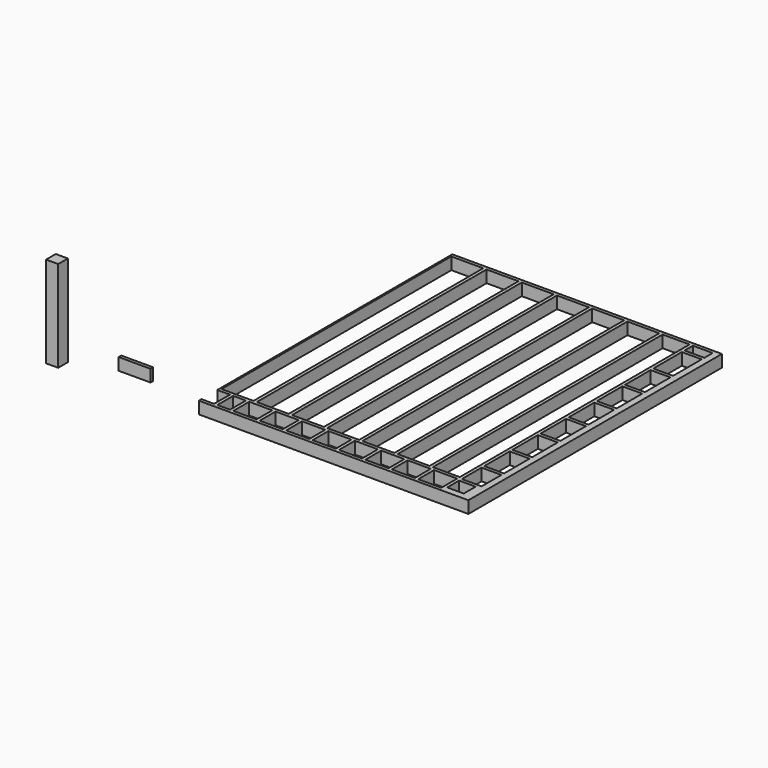
from build123d import *

# Parameters (mm, degrees)
F0_W     = 146.05
F0_H     = 228.6
F0_W_2   = 266.7
F0_W_3   = 190.5
F0_H_2   = 171.45
F0_W_4   = 228.6
F0_H_3   = 368.3
F0_W_5   = 368.3
F0_H_4   = 3314.7
F0_W_6   = 311.15
F0_H_5   = 412.75
F0_H_6   = 120.65
F1_DEPTH = 139.7
F2_W     = 139.7
F2_H     = 139.7
F3_DEPTH = 1054.1
F4_W     = 368.3
F4_H     = 139.7
F5_DEPTH = 38.1


# Not quite as in the source:
# - a feature names something its author has since deleted; it is built from what else it names


with BuildPart() as f1:
    # F0 (on Top) → F1 (new body)
    with BuildSketch(Plane.XY):
        Polygon((403.5037457943, 3406.0115362167), (-2669.8962542057, 3406.0115362167), (-2669.8962542057, 3367.9115362167), (-2669.8962542057, 53.2115362167), (-2669.8962542057, 15.1115362167), (-2523.8462542057, 15.1115362167), (-2523.8462542057, -213.4884637833), (-2669.8962542057, -213.4884637833), (-2669.8962542057, -251.5884637833), (403.5037457943, -251.5884637833), (441.6037457943, -251.5884637833), (441.6037457943, 3406.0115362167), align=None)
        with Locations((-2412.7212542057, -99.1884637833)):
            Rectangle(F0_W, F0_H, mode=Mode.SUBTRACT)
        with Locations((-2168.2462542057, -99.1884637833)):
            Rectangle(F0_W_2, F0_H, mode=Mode.SUBTRACT)
        with Locations((-1863.4462542057, -99.1884637833)):
            Rectangle(F0_W_2, F0_H, mode=Mode.SUBTRACT)
        with Locations((-1558.6462542057, -99.1884637833)):
            Rectangle(F0_W_2, F0_H, mode=Mode.SUBTRACT)
        with Locations((-1253.8462542057, -99.1884637833)):
            Rectangle(F0_W_2, F0_H, mode=Mode.SUBTRACT)
        with Locations((-949.0462542057, -99.1884637833)):
            Rectangle(F0_W_2, F0_H, mode=Mode.SUBTRACT)
        with Locations((-644.2462542057, -99.1884637833)):
            Rectangle(F0_W_2, F0_H, mode=Mode.SUBTRACT)
        with Locations((-339.4462542057, -99.1884637833)):
            Rectangle(F0_W_2, F0_H, mode=Mode.SUBTRACT)
        with Locations((-34.6462542057, -99.1884637833)):
            Rectangle(F0_W_2, F0_H, mode=Mode.SUBTRACT)
        with Locations((232.0537457943, -89.6634637833)):
            Rectangle(F0_W_3, F0_H_2, mode=Mode.SUBTRACT)
        Polygon((365.4037457943, 319.9115362167), (365.4037457943, 65.9115362167), (365.4037457943, 53.2115362167), (365.4037457943, 34.1615362167), (136.8037457943, 34.1615362167), (136.8037457943, 53.2115362167), (136.8037457943, 65.9115362167), (136.8037457943, 319.9115362167), align=None, mode=Mode.SUBTRACT)
        with Locations((251.1037457943, 542.1615362167)):
            Rectangle(F0_W_4, F0_H_3, mode=Mode.SUBTRACT)
        with Locations((251.1037457943, 948.5615362167)):
            Rectangle(F0_W_4, F0_H_3, mode=Mode.SUBTRACT)
        with Locations((251.1037457943, 1354.9615362167)):
            Rectangle(F0_W_4, F0_H_3, mode=Mode.SUBTRACT)
        with Locations((-2466.6962542057, 1710.5615362167)):
            Rectangle(F0_W_5, F0_H_4, mode=Mode.SUBTRACT)
        with Locations((-2060.2962542057, 1710.5615362167)):
            Rectangle(F0_W_5, F0_H_4, mode=Mode.SUBTRACT)
        with Locations((-1653.8962542057, 1710.5615362167)):
            Rectangle(F0_W_5, F0_H_4, mode=Mode.SUBTRACT)
        with Locations((-1247.4962542057, 1710.5615362167)):
            Rectangle(F0_W_5, F0_H_4, mode=Mode.SUBTRACT)
        with Locations((-841.0962542057, 1710.5615362167)):
            Rectangle(F0_W_5, F0_H_4, mode=Mode.SUBTRACT)
        with Locations((-434.6962542057, 1710.5615362167)):
            Rectangle(F0_W_5, F0_H_4, mode=Mode.SUBTRACT)
        with Locations((-56.8712542057, 1710.5615362167)):
            Rectangle(F0_W_6, F0_H_4, mode=Mode.SUBTRACT)
        with Locations((251.1037457943, 1761.3615362167)):
            Rectangle(F0_W_4, F0_H_3, mode=Mode.SUBTRACT)
        with Locations((251.1037457943, 2167.7615362167)):
            Rectangle(F0_W_4, F0_H_3, mode=Mode.SUBTRACT)
        with Locations((251.1037457943, 2574.1615362167)):
            Rectangle(F0_W_4, F0_H_3, mode=Mode.SUBTRACT)
        with Locations((251.1037457943, 3002.7865362167)):
            Rectangle(F0_W_4, F0_H_5, mode=Mode.SUBTRACT)
        with Locations((251.1037457943, 3307.5865362167)):
            Rectangle(F0_W_4, F0_H_6, mode=Mode.SUBTRACT)
    extrude(amount=F1_DEPTH)


with BuildPart() as f3:
    # F2 (on Top) → F3 (new body)
    with BuildSketch(Plane.XY):
        with Locations((-4297.1385696411, -263.3159734249)):
            Rectangle(F2_W, F2_H)
    extrude(amount=F3_DEPTH)


with BuildPart() as f5:
    # F4 (on Front) → F5 (new body)
    with BuildSketch(Plane.XZ):
        with Locations((-3581.8121238708, 69.85)):
            Rectangle(F4_W, F4_H)
    extrude(amount=F5_DEPTH)


solid = Compound([f1.part, f3.part, f5.part])
